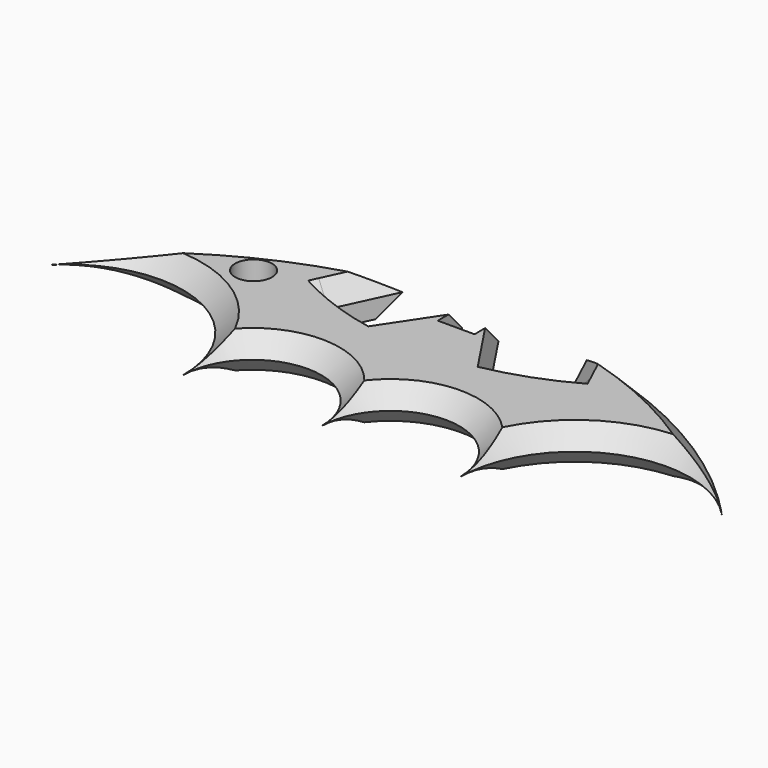
from build123d import *

# Parameters (mm, degrees)
F0_R          = 2
F1_DEPTH      = 4
F2_C1_SIZE    = 2
F2_C2_SIZE    = 1.9999
F2_C3_SIZE    = 2
F2_C4_SIZE    = 2
F2_C5_SIZE    = 2
F2_C6_SIZE    = 1.9999
F2_C7_SIZE    = 2
F2_C8_SIZE    = 1.9999
F2_C9_SIZE    = 2
F2_C10_SIZE   = 1.9999
F2_C11_SIZE   = 2
F2_C12_SIZE   = 1.9999
F2_C13_SIZE   = 2
F2_C14_SIZE   = 1.9999
F3_T4_ANGLE   = 23.1676243984
F3_T9_ANGLE   = 33.0601284412
F3_T15_ANGLE  = 23.1676243984
F3_T20_ANGLE  = 33.0601284412
F3_T26_DEPTH  = 18.3593154951
F3_S27_R      = 30
F3_T28_DEPTH  = 11
F3_T32_DEPTH  = 18.3593154951
F3_S33_R      = 30
F3_T34_DEPTH  = 12
F3_T38_DEPTH  = 18.3593154951
F3_S39_R      = 30
F3_T40_DEPTH  = 11
F3_T44_DEPTH  = 18.3593154951
F3_S45_R      = 30
F3_T46_DEPTH  = 11
F3_T50_ANGLE  = 13.7165010336
F3_T55_ANGLE  = 13.7165010336
F3_T61_ANGLE  = 23.1676243984
F3_T65_DEPTH  = 18.3593154951
F3_S66_R      = 30
F3_T67_DEPTH  = 11
F3_T73_ANGLE  = 33.0601284412
F3_T77_DEPTH  = 18.3593154951
F3_S78_R      = 30
F3_T79_DEPTH  = 12
F3_T85_ANGLE  = 23.1676243984
F3_T89_DEPTH  = 18.3593154951
F3_S90_R      = 30
F3_T91_DEPTH  = 11
F3_T97_ANGLE  = 33.0601284412
F3_T101_DEPTH = 18.3593154951
F3_S102_R     = 30
F3_T103_DEPTH = 11


# Not quite as in the source:
# - a fillet or chamfer that OpenCascade refuses, or shapes differently, is made with other operations: its cross-section is extruded or revolved along the edge and cut away or added
# - a fillet or chamfer is up to 0.001 mm smaller than in the source, because OpenCascade refuses the exact size


with BuildPart() as f1:
    # F0 (on Top) → F1 (new body)
    with BuildSketch(Plane.XY):
        with BuildLine():
            Line((-12.9583278322, 42.6456403464), (-10, 48.9897948557))
            ThreePointArc((-10, 48.9897948557), (-24.5085073708, 43.5813385115), (-36.6666666667, 33.993463424))
            ThreePointArc((-36.6666666667, 33.993463424), (-22.9356453541, 37.1319642711), (-15, 25.495097568))
            ThreePointArc((-15, 25.495097568), (-7.5, 32.995097568), (0, 25.495097568))
            ThreePointArc((0, 25.495097568), (7.5, 32.995097568), (15, 25.495097568))
            ThreePointArc((15, 25.495097568), (22.9356453541, 37.1319642711), (36.6666666667, 33.993463424))
            ThreePointArc((36.6666666667, 33.993463424), (24.5085073708, 43.5813385115), (10, 48.9897948557))
            Line((10, 48.9897948557), (12.9583278322, 42.6456403464))
            ThreePointArc((12.9583278322, 42.6456403464), (9.7439963261, 41.3291664505), (6.3990408051, 40.3930558198))
            ThreePointArc((6.3990408051, 40.3930558198), (0, 39.702649416), (-6.3990408051, 40.3930558198))
            ThreePointArc((-6.3990408051, 40.3930558198), (-9.7439963261, 41.3291664505), (-12.9583278322, 42.6456403464))
        make_face()
        with Locations((-19.9469160289, 41.2377901375)):
            Circle(F0_R, mode=Mode.SUBTRACT)
        with BuildLine():
            Line((-1.9713696092, 47.056067735), (-6.3990408051, 40.3930558198))
            ThreePointArc((-6.3990408051, 40.3930558198), (0, 39.702649416), (6.3990408051, 40.3930558198))
            Line((6.3990408051, 40.3930558198), (1.9713696092, 47.056067735))
            Line((1.9713696092, 47.056067735), (2, 43.7767133248))
            Line((2, 43.7767133248), (0, 43.7767133248))
            Line((0, 43.7767133248), (-2, 43.7767133248))
            Line((-2, 43.7767133248), (-1.9713696092, 47.056067735))
        make_face()
    extrude(amount=F1_DEPTH)

    # F2: chamfer of 2 on 14 edges, made by hand

    # F2_c1
    f2_c1_edges = [f1.edges().sort_by_distance(p)[0] for p in [
        (24.5085073708, 43.5813385115, 0),
    ]]
    chamfer(f2_c1_edges, length=F2_C1_SIZE)

    # F2_c2 (size 2 in the source; OpenCascade refuses exactly that, so slightly less here)
    f2_c2_edges = [f1.edges().sort_by_distance(p)[0] for p in [
        (24.5085073708, 43.5813385115, 4),
    ]]
    chamfer(f2_c2_edges, length=F2_C2_SIZE)

    # F2_c3
    f2_c3_edges = [f1.edges().sort_by_distance(p)[0] for p in [
        (12.011285826, 44.6765784827, 4),
    ]]
    chamfer(f2_c3_edges, length=F2_C3_SIZE)

    # F2_c4
    f2_c4_edges = [f1.edges().sort_by_distance(p)[0] for p in [
        (-11.4791639161, 45.817717601, 4),
    ]]
    chamfer(f2_c4_edges, length=F2_C4_SIZE)

    # F2_c5
    f2_c5_edges = [f1.edges().sort_by_distance(p)[0] for p in [
        (-24.5085073708, 43.5813385115, 0),
    ]]
    chamfer(f2_c5_edges, length=F2_C5_SIZE)

    # F2_c6 (size 2 in the source; OpenCascade refuses exactly that, so slightly less here)
    f2_c6_edges = [f1.edges().sort_by_distance(p)[0] for p in [
        (-25.6065907207, 42.9453433059, 4),
    ]]
    chamfer(f2_c6_edges, length=F2_C6_SIZE)

    # F2_c7
    f2_c7_edges = [f1.edges().sort_by_distance(p)[0] for p in [
        (-19.4184053045, 35.031230284, 0),
    ]]
    chamfer(f2_c7_edges, length=F2_C7_SIZE)

    # F2_c8 (size 2 in the source; OpenCascade refuses exactly that, so slightly less here)
    f2_c8_edges = [f1.edges().sort_by_distance(p)[0] for p in [
        (-19.4184850979, 35.031297906, 4),
    ]]
    chamfer(f2_c8_edges, length=F2_C8_SIZE)

    # F2_c9
    f2_c9_edges = [f1.edges().sort_by_distance(p)[0] for p in [
        (-5.25, 32.6496415786, 0),
    ]]
    chamfer(f2_c9_edges, length=F2_C9_SIZE)

    # F2_c10 (size 2 in the source; OpenCascade refuses exactly that, so slightly less here)
    f2_c10_edges = [f1.edges().sort_by_distance(p)[0] for p in [
        (-5.2500604173, 32.6496605787, 4),
    ]]
    chamfer(f2_c10_edges, length=F2_C10_SIZE)

    # F2_c11
    f2_c11_edges = [f1.edges().sort_by_distance(p)[0] for p in [
        (9.5615528128, 32.7062001189, 0),
    ]]
    chamfer(f2_c11_edges, length=F2_C11_SIZE)

    # F2_c12 (size 2 in the source; OpenCascade refuses exactly that, so slightly less here)
    f2_c12_edges = [f1.edges().sort_by_distance(p)[0] for p in [
        (9.5614952101, 32.7062165864, 4),
    ]]
    chamfer(f2_c12_edges, length=F2_C12_SIZE)

    # F2_c13
    f2_c13_edges = [f1.edges().sort_by_distance(p)[0] for p in [
        (21.3153564799, 36.3578865528, 0),
    ]]
    chamfer(f2_c13_edges, length=F2_C13_SIZE)

    # F2_c14 (size 2 in the source; OpenCascade refuses exactly that, so slightly less here)
    f2_c14_edges = [f1.edges().sort_by_distance(p)[0] for p in [
        (21.3153904307, 36.3579058824, 4),
    ]]
    chamfer(f2_c14_edges, length=F2_C14_SIZE)

    # F3: chamfer of 2 x 1 on 8 edges, made by hand


with BuildPart() as f3_tool2:
    # F3_s3 → F3_t4 (revolve)
    with BuildSketch(Plane(origin=(-2.9446339923, 0.1246207965, 0), x_dir=(0, 0, 1), z_dir=(0.9991056542, -0.0422834698, 0))):
        Polygon((4, -38.6403111418), (2, -39.6403111418), (4, -39.6403111418), align=None)
    revolve(axis=Axis((0, 69.702649416, 4), (0, 0, -1)), revolution_arc=F3_T4_ANGLE)

    split(bisect_by=Plane(origin=(-23.0586077624, 15.3227901596, 0), x_dir=(0, 0, 1), z_dir=(-0.8328764894, 0.5534588995, 0)), keep=Keep.TOP)


with BuildPart() as f1_1:
    add(f1.part)

    # F3_t1: cut F3_tool2
    add(f3_tool2.part, mode=Mode.SUBTRACT)


with BuildPart() as f3_tool7:
    # F3_s8 → F3_t9 (revolve)
    with BuildSketch(Plane(origin=(-2.9446339923, 0.1246207965, 0), x_dir=(0, 0, 1), z_dir=(0.9991056542, -0.0422834698, 0))):
        Polygon((0, -38.6403111418), (2, -39.6403111418), (0, -39.6403111418), align=None)
    revolve(axis=Axis((0, 69.702649416, 0), (0, 0, -1)), revolution_arc=F3_T9_ANGLE)

    split(bisect_by=Plane(origin=(-23.0586077624, 15.3227901596, 0), x_dir=(0, 0, 1), z_dir=(-0.8328764894, 0.5534588995, 0)), keep=Keep.TOP)

    split(bisect_by=Plane(origin=(-26.9781181078, 12.5801030763, 0), x_dir=(0, 0, 1), z_dir=(0.906307787, -0.4226182617, 0)), keep=Keep.TOP)


with BuildPart() as f1_2:
    add(f1_1.part)

    # F3_t6: cut F3_tool7
    add(f3_tool7.part, mode=Mode.SUBTRACT)


with BuildPart() as f3_tool13:
    # F3_s14 → F3_t15 (revolve)
    with BuildSketch(Plane(origin=(27.1541071122, 13.0048306908, 0), x_dir=(0, 0, 1), z_dir=(0.9019003023, 0.4319442611, 0))):
        Polygon((4, -31.8648405809), (2, -32.8648405809), (4, -32.8648405809), align=None)
    revolve(axis=Axis((0, 69.702649416, 4), (0, 0, -1)), revolution_arc=F3_T15_ANGLE)

    split(bisect_by=Plane(origin=(23.0586077624, 15.3227901596, 0), x_dir=(0, 0, 1), z_dir=(0.8328764894, 0.5534588995, 0)), keep=Keep.TOP)


with BuildPart() as f1_3:
    add(f1_2.part)

    # F3_t12: cut F3_tool13
    add(f3_tool13.part, mode=Mode.SUBTRACT)


with BuildPart() as f3_tool18:
    # F3_s19 → F3_t20 (revolve)
    with BuildSketch(Plane(origin=(32.9460403942, 23.4858833946, 0), x_dir=(0, 0, 1), z_dir=(0.8142825601, 0.5804687006, 0))):
        Polygon((0, -24.7576518113), (1, -26.7576518113), (0, -26.7576518113), align=None)
    revolve(axis=Axis((0, 69.702649416, 0), (0, 0, -1)), revolution_arc=F3_T20_ANGLE)

    split(bisect_by=Plane(origin=(23.0586077624, 15.3227901596, 0), x_dir=(0, 0, 1), z_dir=(0.8328764894, 0.5534588995, 0)), keep=Keep.TOP)

    split(bisect_by=Plane(origin=(26.9781181078, 12.5801030763, 0), x_dir=(0, 0, 1), z_dir=(-0.906307787, -0.4226182617, 0)), keep=Keep.TOP)


with BuildPart() as f1_4:
    add(f1_3.part)

    # F3_t17: cut F3_tool18
    add(f3_tool18.part, mode=Mode.SUBTRACT)


with BuildPart() as f3_tool24:
    # F3_s25 → F3_t26 (new body)
    with BuildSketch(Plane(origin=(23.9539658298, 36.0472927364, 0), x_dir=(0, 0, 1), z_dir=(-0.5534588995, -0.8328764894, 0))):
        Polygon((4, 26.6855068621), (2, 27.6855068621), (4, 27.6855068621), align=None)
    extrude(amount=F3_T26_DEPTH)

    # F3_s27 → F3_t28 (intersect, symmetric)
    with BuildSketch(Plane.XY.offset(3)):
        with Locations((0, 69.702649416)):
            Circle(F3_S27_R)
    extrude(amount=F3_T28_DEPTH, both=True, mode=Mode.INTERSECT)


with BuildPart() as f1_5:
    add(f1_4.part)

    # F3_t23: cut F3_tool24
    add(f3_tool24.part, mode=Mode.SUBTRACT)


with BuildPart() as f3_tool30:
    # F3_s31 → F3_t32 (new body)
    with BuildSketch(Plane(origin=(23.9539658298, 36.0472927364, 0), x_dir=(0, 0, 1), z_dir=(-0.5534588995, -0.8328764894, 0))):
        Polygon((0, 25.6855068621), (1, 27.6855068621), (0, 27.6855068621), align=None)
    extrude(amount=F3_T32_DEPTH)

    # F3_s33 → F3_t34 (intersect, symmetric)
    with BuildSketch(Plane.XY.offset(0.5)):
        with Locations((0, 69.702649416)):
            Circle(F3_S33_R)
    extrude(amount=F3_T34_DEPTH, both=True, mode=Mode.INTERSECT)


with BuildPart() as f1_6:
    add(f1_5.part)

    # F3_t29: cut F3_tool30
    add(f3_tool30.part, mode=Mode.SUBTRACT)


with BuildPart() as f3_tool36:
    # F3_s37 → F3_t38 (new body)
    with BuildSketch(Plane(origin=(-13.7928392805, 20.7562504992, 0), x_dir=(0, 0, 1), z_dir=(-0.5534588995, 0.8328764894, 0))):
        Polygon((4, 26.6855068621), (2, 27.6855068621), (4, 27.6855068621), align=None)
    extrude(amount=F3_T38_DEPTH)

    # F3_s39 → F3_t40 (intersect, symmetric)
    with BuildSketch(Plane.XY.offset(3)):
        with Locations((0, 69.702649416)):
            Circle(F3_S39_R)
    extrude(amount=F3_T40_DEPTH, both=True, mode=Mode.INTERSECT)


with BuildPart() as f1_7:
    add(f1_6.part)

    # F3_t35: cut F3_tool36
    add(f3_tool36.part, mode=Mode.SUBTRACT)


with BuildPart() as f3_tool42:
    # F3_s43 → F3_t44 (new body)
    with BuildSketch(Plane(origin=(-13.7928392805, 20.7562504992, 0), x_dir=(0, 0, 1), z_dir=(-0.5534588995, 0.8328764894, 0))):
        Polygon((0, 26.6855068621), (2, 27.6855068621), (0, 27.6855068621), align=None)
    extrude(amount=F3_T44_DEPTH)

    # F3_s45 → F3_t46 (intersect, symmetric)
    with BuildSketch(Plane.XY.offset(1)):
        with Locations((0, 69.702649416)):
            Circle(F3_S45_R)
    extrude(amount=F3_T46_DEPTH, both=True, mode=Mode.INTERSECT)


with BuildPart() as f1_8:
    add(f1_7.part)

    # F3_t41: cut F3_tool42
    add(f3_tool42.part, mode=Mode.SUBTRACT)


with BuildPart() as f3_tool48:
    # F3_s49 → F3_t50 (revolve)
    with BuildSketch(Plane(origin=(27.1541071122, 13.0048306908, 0), x_dir=(0, 0, 1), z_dir=(-0.9019003023, -0.4319442611, 0))):
        Polygon((4, 31.8648405809), (2, 32.8648405809), (4, 32.8648405809), align=None)
    revolve(axis=Axis((0, 69.702649416, 4), (0, 0, 1)), revolution_arc=F3_T50_ANGLE)

    split(bisect_by=Plane(origin=(12.5827512669, 5.8674332764, -13.8835299077), x_dir=(0.4226182617, -0.906307787, 0), z_dir=(-0.6408563821, -0.2988362387, 0.7071067812)), keep=Keep.TOP)


with BuildPart() as f1_9:
    add(f1_8.part)

    # F3_t47: cut F3_tool48
    add(f3_tool48.part, mode=Mode.SUBTRACT)


with BuildPart() as f3_tool53:
    # F3_s54 → F3_t55 (revolve)
    with BuildSketch(Plane(origin=(-27.1541071122, 13.0048306908, 0), x_dir=(0, 0, 1), z_dir=(0.9019003023, -0.4319442611, 0))):
        Polygon((4, -31.8648405809), (2, -32.8648405809), (4, -32.8648405809), align=None)
    revolve(axis=Axis((0, 69.702649416, 4), (0, 0, -1)), revolution_arc=F3_T55_ANGLE)

    split(bisect_by=Plane(origin=(-12.5827512669, 5.8674332764, -13.8835299077), x_dir=(0.4226182617, 0.906307787, 0), z_dir=(0.6408563821, -0.2988362387, 0.7071067812)), keep=Keep.TOP)


with BuildPart() as f1_10:
    add(f1_9.part)

    # F3_t52: cut F3_tool53
    add(f3_tool53.part, mode=Mode.SUBTRACT)


with BuildPart() as f3_tool59:
    # F3_s60 → F3_t61 (revolve)
    with BuildSketch(Plane(origin=(-2.9446339923, 0.1246207965, 0), x_dir=(0, 0, 1), z_dir=(0.9991056542, -0.0422834698, 0))):
        Polygon((4, -38.6403111418), (2, -39.6403111418), (4, -39.6403111418), align=None)
    revolve(axis=Axis((0, 69.702649416, 4), (0, 0, -1)), revolution_arc=F3_T61_ANGLE)

    split(bisect_by=Plane(origin=(-23.0586077624, 15.3227901596, 0), x_dir=(0, 0, 1), z_dir=(0.8328764894, -0.5534588995, 0)), keep=Keep.TOP)


with BuildPart() as f3_tool63:
    # F3_s64 → F3_t65 (new body)
    with BuildSketch(Plane(origin=(23.9539658298, 36.0472927364, 0), x_dir=(0, 0, 1), z_dir=(-0.5534588995, -0.8328764894, 0))):
        Polygon((4, 26.6855068621), (2, 27.6855068621), (4, 27.6855068621), align=None)
    extrude(amount=F3_T65_DEPTH)

    # F3_s66 → F3_t67 (cut, symmetric)
    with BuildSketch(Plane.XY.offset(3)):
        with Locations((0, 69.702649416)):
            Circle(F3_S66_R)
    extrude(amount=F3_T67_DEPTH, both=True, mode=Mode.SUBTRACT)


with BuildPart() as f3_tool59_1:
    add(f3_tool59.part)

    # F3_t68: intersect F3_tool63
    add(f3_tool63.part, mode=Mode.INTERSECT)


with BuildPart() as f1_11:
    add(f1_10.part)

    # F3_t57: cut F3_tool59
    add(f3_tool59_1.part, mode=Mode.SUBTRACT)


with BuildPart() as f3_tool71:
    # F3_s72 → F3_t73 (revolve)
    with BuildSketch(Plane(origin=(-2.9446339923, 0.1246207965, 0), x_dir=(0, 0, 1), z_dir=(0.9991056542, -0.0422834698, 0))):
        Polygon((0, -38.6403111418), (2, -39.6403111418), (0, -39.6403111418), align=None)
    revolve(axis=Axis((0, 69.702649416, 0), (0, 0, -1)), revolution_arc=F3_T73_ANGLE)

    split(bisect_by=Plane(origin=(-23.0586077624, 15.3227901596, 0), x_dir=(0, 0, 1), z_dir=(0.8328764894, -0.5534588995, 0)), keep=Keep.TOP)


with BuildPart() as f3_tool75:
    # F3_s76 → F3_t77 (new body)
    with BuildSketch(Plane(origin=(23.9539658298, 36.0472927364, 0), x_dir=(0, 0, 1), z_dir=(-0.5534588995, -0.8328764894, 0))):
        Polygon((0, 25.6855068621), (1, 27.6855068621), (0, 27.6855068621), align=None)
    extrude(amount=F3_T77_DEPTH)

    # F3_s78 → F3_t79 (cut, symmetric)
    with BuildSketch(Plane.XY.offset(0.5)):
        with Locations((0, 69.702649416)):
            Circle(F3_S78_R)
    extrude(amount=F3_T79_DEPTH, both=True, mode=Mode.SUBTRACT)


with BuildPart() as f3_tool71_1:
    add(f3_tool71.part)

    # F3_t80: intersect F3_tool75
    add(f3_tool75.part, mode=Mode.INTERSECT)


with BuildPart() as f1_12:
    add(f1_11.part)

    # F3_t69: cut F3_tool71
    add(f3_tool71_1.part, mode=Mode.SUBTRACT)


with BuildPart() as f3_tool83:
    # F3_s84 → F3_t85 (revolve)
    with BuildSketch(Plane(origin=(27.1541071122, 13.0048306908, 0), x_dir=(0, 0, 1), z_dir=(0.9019003023, 0.4319442611, 0))):
        Polygon((4, -31.8648405809), (2, -32.8648405809), (4, -32.8648405809), align=None)
    revolve(axis=Axis((0, 69.702649416, 4), (0, 0, -1)), revolution_arc=F3_T85_ANGLE)

    split(bisect_by=Plane(origin=(23.0586077624, 15.3227901596, 0), x_dir=(0, 0, 1), z_dir=(-0.8328764894, -0.5534588995, 0)), keep=Keep.TOP)


with BuildPart() as f3_tool87:
    # F3_s88 → F3_t89 (new body)
    with BuildSketch(Plane(origin=(-13.7928392805, 20.7562504992, 0), x_dir=(0, 0, 1), z_dir=(-0.5534588995, 0.8328764894, 0))):
        Polygon((4, 26.6855068621), (2, 27.6855068621), (4, 27.6855068621), align=None)
    extrude(amount=F3_T89_DEPTH)

    # F3_s90 → F3_t91 (cut, symmetric)
    with BuildSketch(Plane.XY.offset(3)):
        with Locations((0, 69.702649416)):
            Circle(F3_S90_R)
    extrude(amount=F3_T91_DEPTH, both=True, mode=Mode.SUBTRACT)


with BuildPart() as f3_tool83_1:
    add(f3_tool83.part)

    # F3_t92: intersect F3_tool87
    add(f3_tool87.part, mode=Mode.INTERSECT)


with BuildPart() as f1_13:
    add(f1_12.part)

    # F3_t81: cut F3_tool83
    add(f3_tool83_1.part, mode=Mode.SUBTRACT)


with BuildPart() as f3_tool95:
    # F3_s96 → F3_t97 (revolve)
    with BuildSketch(Plane(origin=(32.9460403942, 23.4858833946, 0), x_dir=(0, 0, 1), z_dir=(0.8142825601, 0.5804687006, 0))):
        Polygon((0, -24.7576518113), (1, -26.7576518113), (0, -26.7576518113), align=None)
    revolve(axis=Axis((0, 69.702649416, 0), (0, 0, -1)), revolution_arc=F3_T97_ANGLE)

    split(bisect_by=Plane(origin=(23.0586077624, 15.3227901596, 0), x_dir=(0, 0, 1), z_dir=(-0.8328764894, -0.5534588995, 0)), keep=Keep.TOP)


with BuildPart() as f3_tool99:
    # F3_s100 → F3_t101 (new body)
    with BuildSketch(Plane(origin=(-13.7928392805, 20.7562504992, 0), x_dir=(0, 0, 1), z_dir=(-0.5534588995, 0.8328764894, 0))):
        Polygon((0, 26.6855068621), (2, 27.6855068621), (0, 27.6855068621), align=None)
    extrude(amount=F3_T101_DEPTH)

    # F3_s102 → F3_t103 (cut, symmetric)
    with BuildSketch(Plane.XY.offset(1)):
        with Locations((0, 69.702649416)):
            Circle(F3_S102_R)
    extrude(amount=F3_T103_DEPTH, both=True, mode=Mode.SUBTRACT)


with BuildPart() as f3_tool95_1:
    add(f3_tool95.part)

    # F3_t104: intersect F3_tool99
    add(f3_tool99.part, mode=Mode.INTERSECT)


with BuildPart() as f1_14:
    add(f1_13.part)

    # F3_t93: cut F3_tool95
    add(f3_tool95_1.part, mode=Mode.SUBTRACT)


solid = f1_14.part
